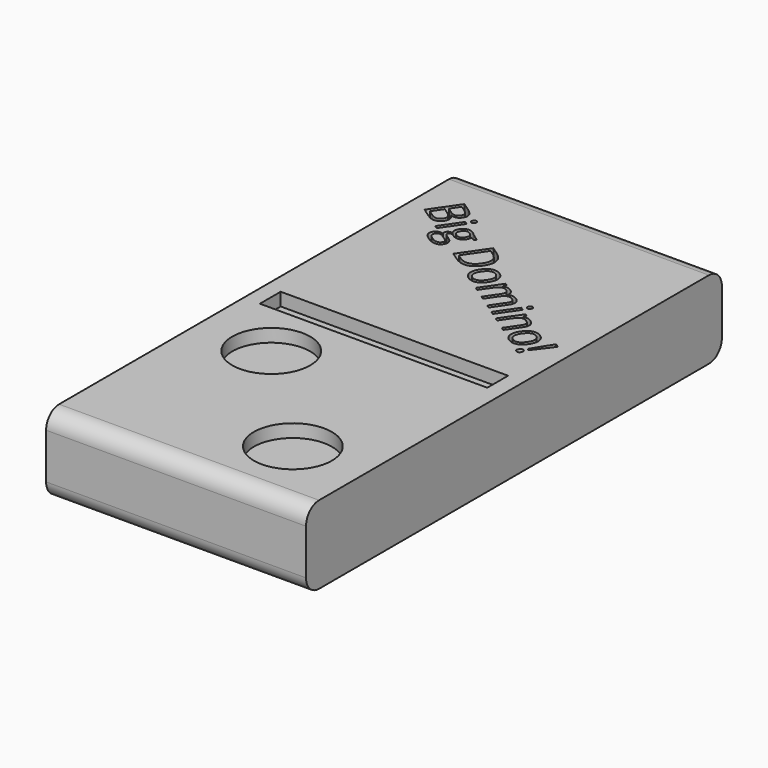
from build123d import *

# Parameters (mm, degrees)
F0_W         = 50.8
F0_H         = 101.6
F1_DEPTH     = 15.24
F2_R         = 3.175
F3_W         = 44.45
F3_H         = 5.08
F3_R         = 7.62
F3_TEXT_SIZE = 8.9132580327
F4_DEPTH     = 2.54


# Not quite as in the source:
# - Text() gives the source's letters only with a copy of the font that has no kerning and outlines rounded to 1/6400 em; it was checked with that copy


with BuildPart() as f1:
    # F0 (on Top) → F1 (new body)
    with BuildSketch(Plane.XY):
        Rectangle(F0_W, F0_H)
    extrude(amount=F1_DEPTH)

    # F2
    f2_edges = [f1.edges().sort_by_distance(p)[0] for p in [
        (0, -50.8, 15.24),
        (0, -50.8, 0),
        (0, 50.8, 15.24),
        (0, 50.8, 0),
    ]]
    fillet(f2_edges, radius=F2_R)

    # F3 (on face) → F4 (cut)
    with BuildSketch(Plane.XY.offset(15.24)):
        Rectangle(F3_W, F3_H)
        with Locations((-11.1125, -13.6525)):
            Circle(F3_R)
        with Locations((11.1441062763, -36.195)):
            Circle(F3_R)
        with Locations(Location((-22.7420448029, 37.9251808441), (0, 0, -34.5401274845))):
            Text('Big Domino!', F3_TEXT_SIZE, font='Open Sans', text_align=(TextAlign.LEFT, TextAlign.BOTTOM))
    extrude(amount=-F4_DEPTH, mode=Mode.SUBTRACT)


solid = f1.part
